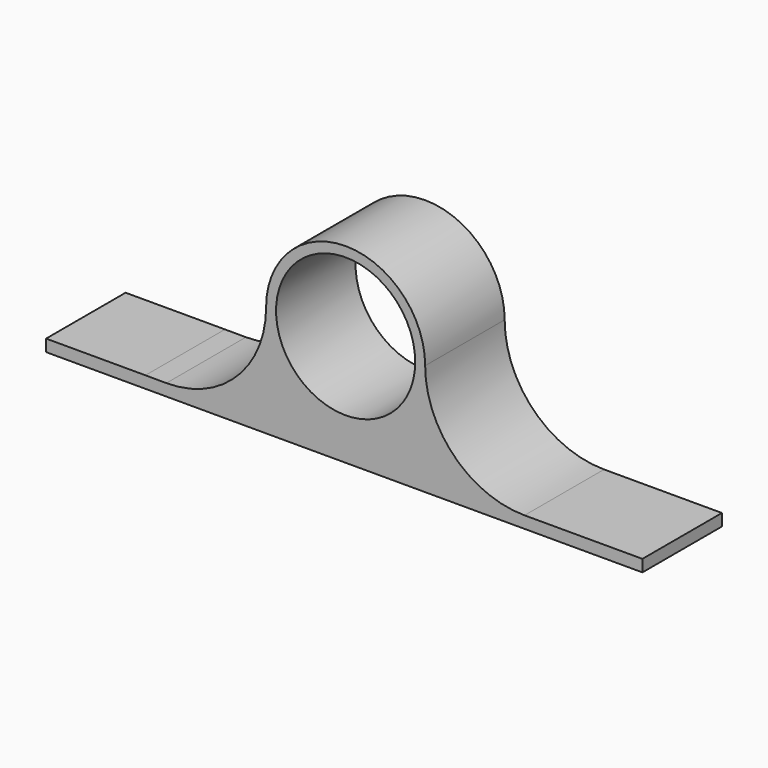
from build123d import *

# Parameters (mm, degrees)
F0_R     = 17.5
F1_DEPTH = 25


# Not quite as in the source:
# - ends of sketch curves that miss each other by under 0.0002 mm in the source are joined


with BuildPart() as f1:
    # F0 (on Front) → F1 (new body)
    with BuildSketch(Plane.XZ):
        with BuildLine():
            ThreePointArc((45, -25), (27.3223304703, -17.6776695297), (20, 0))
            ThreePointArc((20, 0), (0.0107860663, -19.9999970915), (-19.9999883661, -0.0215721294))
            ThreePointArc((-19.9999883661, -0.0215721294), (-27.3583172251, -17.7351553161), (-45.1016823096, -25.0213653552))
            Line((-45.1016823096, -25.0213653552), (-50.3546064898, -25))
            Line((-50.3546064898, -25), (-75.3500018494, -25))
            Line((-75.3500018494, -25), (-75.3500018494, -28))
            Line((-75.3500018494, -28), (74.6500011308, -28))
            Line((74.6500011308, -28), (74.65, -25))
            Line((74.65, -25), (50.3546064898, -25))
            Line((50.3546064898, -25), (45, -25))
        make_face()
        with BuildLine():
            ThreePointArc((-19.9999883661, -0.0215721294), (0.0107860663, -19.9999970915), (20, 0))
            ThreePointArc((20, 0), (0, 20), (-20, 0))
            ThreePointArc((-20, 0), (-19.9999970915, -0.0107860663), (-19.9999883661, -0.0215721294))
        make_face()
        Circle(F0_R, mode=Mode.SUBTRACT)
    extrude(amount=F1_DEPTH)


solid = f1.part
